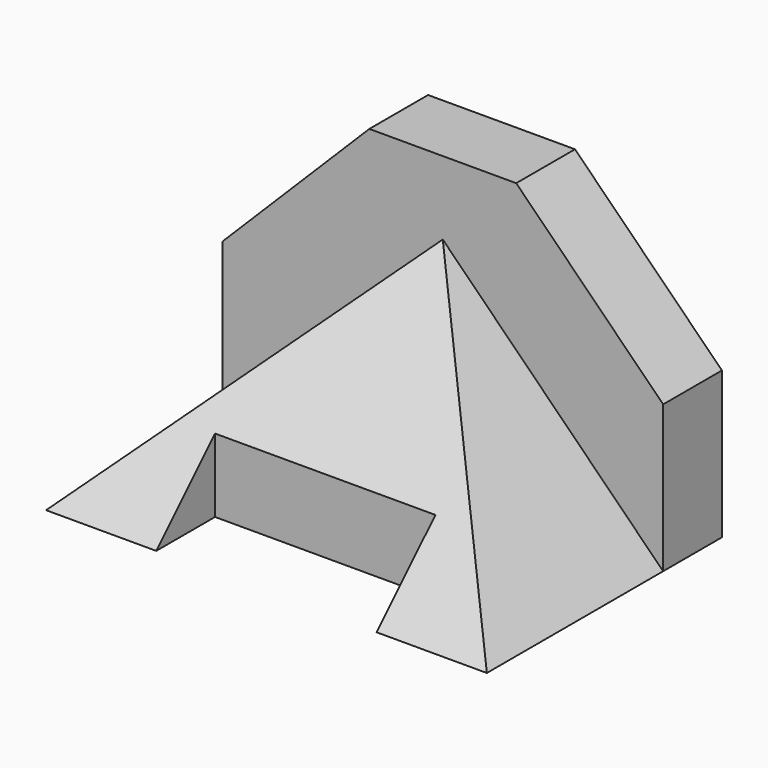
from build123d import *

# Parameters (mm, degrees)
F2_W      = 12.7
F2_H      = 25.4
F3_DEPTH  = 76.2
F4_DEPTH  = 50.801
F6_DEPTH  = 50.8
F7_DEPTH  = 38.1
F8_DEPTH  = 76.2
F9_DEPTH  = 50.801
F11_DEPTH = 155
F13_DEPTH = 76.2
F1_W      = 38.1
F1_H      = 12.7
F14_DEPTH = 12.7


# Not quite as in the source:
# - an extrude ends at something that could not be found from the text; its depth is read off the source's solid


with BuildPart() as f3:
    # F2 (on Right) → F3 (new body)
    with BuildSketch(Plane.YZ):
        Polygon((38.1, 50.8), (38.1, 38.1), (38.1, 25.4), (50.8, 25.4), (50.8, 50.8), align=None)
        with Locations((44.45, 12.7)):
            Rectangle(F2_W, F2_H)
    extrude(amount=F3_DEPTH)

    # F0 (on Front) → F4 (cut, through all)
    with BuildSketch(Plane.XZ):
        Polygon((0, 50.8), (0, 25.4), (25.4, 50.8), align=None)
        Polygon((76.2, 50.8), (50.8, 50.8), (76.2, 25.4), align=None)
    extrude(amount=-F4_DEPTH, mode=Mode.SUBTRACT)


with BuildPart() as f6:
    # F5 (on face) → F6 (new body)
    with BuildSketch(Plane.XY.offset(50.8)):
        Polygon((76.2, 0), (38.1, 38.1), (0, 0), align=None)
    extrude(amount=-F6_DEPTH)

    # F0 (on Front) → F7 (cut, through all)
    with BuildSketch(Plane.XZ):
        Polygon((0, 25.4), (0, 0), (38.1, 38.1), (76.2, 0), (76.2, 25.4), (50.8, 50.8), (25.4, 50.8), align=None)
    extrude(amount=-F7_DEPTH, mode=Mode.SUBTRACT)


with BuildPart() as f8:
    # F2 (on Right) → F8 (new body)
    with BuildSketch(Plane.YZ):
        Polygon((38.1, 38.1), (0, 0), (38.1, 0), (38.1, 25.4), align=None)
    extrude(amount=F8_DEPTH)


with BuildPart() as f9_tool:
    # F9 (cut, through all): faces of the model
    f9_faces = [f6.part.faces().sort_by_distance(p)[0] for p in [
        (67.7333333333, 0, 42.3333333333),
        (8.4666666667, 0, 42.3333333333),
    ]]
    extrude(f9_faces, amount=-F9_DEPTH)


with BuildPart() as f6_1:
    add(f6.part)

    # F9: cut by f9_tool
    add(f9_tool.part, mode=Mode.SUBTRACT)

    # F10 (on face) → F11 (cut, through all)
    with BuildSketch(Plane(origin=(0, 0, 0), x_dir=(1, 0, 0), z_dir=(0, -0.7071067812, 0.7071067812))):
        Polygon((63.5, 53.8815367264), (12.7, 53.8815367264), (0, 35.9210244843), (0, 0), (76.2, 0), (76.2, 35.9210244843), align=None)
    extrude(amount=F11_DEPTH, mode=Mode.SUBTRACT)


with BuildPart() as f8_1:
    add(f8.part)

    # F9: cut by f9_tool
    add(f9_tool.part, mode=Mode.SUBTRACT)

    # F12 (on face) → F13 (cut)
    with BuildSketch(Plane.XZ.offset(-38.1)):
        Polygon((76.2, 38.1), (38.1, 38.1), (76.2, 0), align=None)
        Polygon((0, 0), (38.1, 38.1), (0, 38.1), align=None)
    extrude(amount=F13_DEPTH, mode=Mode.SUBTRACT)


with BuildPart() as f14_tool:
    # F1 (on Top) → F14 (new body)
    with BuildSketch(Plane.XY):
        with Locations((38.1, 6.35)):
            Rectangle(F1_W, F1_H)
    extrude(amount=F14_DEPTH)


with BuildPart() as f6_2:
    add(f6_1.part)

    # F14: cut by f14_tool
    add(f14_tool.part, mode=Mode.SUBTRACT)


with BuildPart() as f8_2:
    add(f8_1.part)

    # F14: cut by f14_tool
    add(f14_tool.part, mode=Mode.SUBTRACT)


solid = Compound([f3.part, f6_2.part, f8_2.part])
